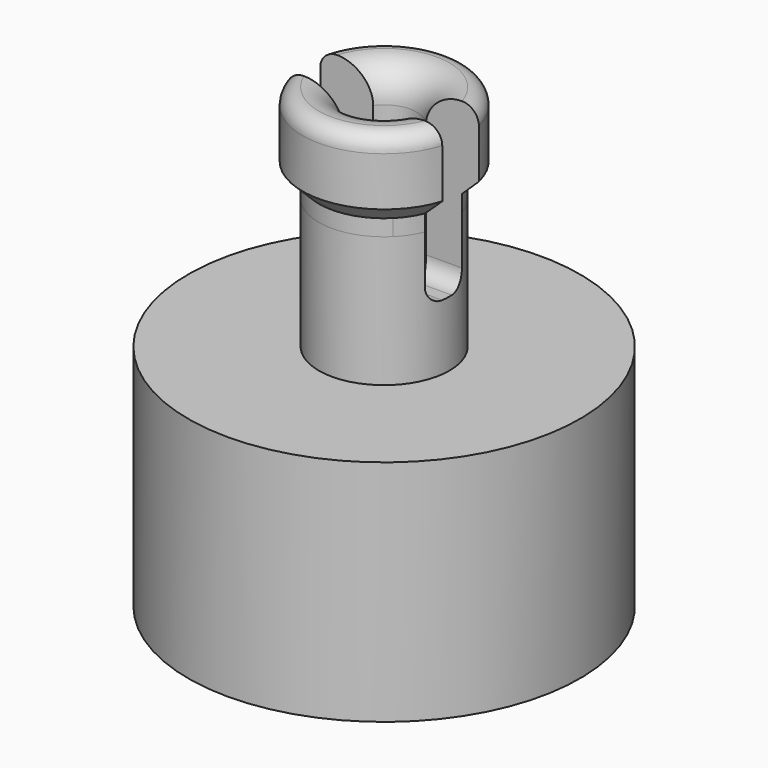
from build123d import *

# Parameters (mm, degrees)
F3_DEPTH     = 5
F4_T4_ANGLE  = 270.6670948428
F4_S5_R      = 2
F4_T6_DEPTH  = 5
F4_T10_ANGLE = 262.8807253971
F4_S11_R     = 2
F4_T12_DEPTH = 5
F5_SIZE      = 1
F6_R         = 1
F7_R         = 0.49999
F8_R         = 0.5
F9_W         = 20.6344220787
F9_H         = 19.8933202773
F9_R         = 5
F10_DEPTH    = 5
F11_R        = 2.8
F12_DEPTH    = 6.4


# Not quite as in the source:
# - a fillet or chamfer that OpenCascade refuses, or shapes differently, is made with other operations: its cross-section is extruded or revolved along the edge and cut away or added
# - a fillet or chamfer is up to 0.001 mm smaller than in the source, because OpenCascade refuses the exact size


with BuildPart() as f1:
    # F0 (on Right) → F1 (revolve)
    with BuildSketch(Plane.YZ):
        Polygon((-6, 0), (0, 0), (0, 12), (-1, 12), (-1, 16), (-1, 19), (-2, 19), (-2.5, 19), (-2.5, 16), (-2, 16), (-2, 12), (-6, 12), align=None)
    revolve(axis=Axis((0, 0, 6), (0, 0, -1)))

    # F2 (on face) → F3 (cut)
    with BuildSketch(Plane.XY.offset(19)):
        with BuildLine():
            Line((-0.8067003414, 0.5909607086), (-2.4291491187, 0.5909607086))
            ThreePointArc((-2.4291491187, 0.5909607086), (-2.4985623215, -0.0847721969), (-2.3835084063, -0.75424643))
            Line((-2.3835084063, -0.75424643), (-0.6565914428, -0.75424643))
            ThreePointArc((-0.6565914428, -0.75424643), (-0.993831612, -0.1108996261), (-0.8067003414, 0.5909607086))
        make_face()
        with BuildLine():
            ThreePointArc((1, 0), (0.9504473529, 0.3108855566), (0.8067003414, 0.5909607086))
            Line((0.8067003414, 0.5909607086), (-0.8067003414, 0.5909607086))
            ThreePointArc((-0.8067003414, 0.5909607086), (-0.993831612, -0.1108996261), (-0.6565914428, -0.75424643))
            Line((-0.6565914428, -0.75424643), (0.6565914428, -0.75424643))
            ThreePointArc((0.6565914428, -0.75424643), (0.9101075329, -0.4143721499), (1, 0))
        make_face()
        with BuildLine():
            ThreePointArc((2.5, 0), (2.482224083, 0.2975963737), (2.4291491187, 0.5909607086))
            Line((2.4291491187, 0.5909607086), (0.8067003414, 0.5909607086))
            ThreePointArc((0.8067003414, 0.5909607086), (0.9504473529, 0.3108855566), (1, 0))
            ThreePointArc((1, 0), (0.9101075329, -0.4143721499), (0.6565914428, -0.75424643))
            Line((0.6565914428, -0.75424643), (2.3835084063, -0.75424643))
            ThreePointArc((2.3835084063, -0.75424643), (2.4707054676, -0.38159467), (2.5, 0))
        make_face()
    extrude(amount=-F3_DEPTH, mode=Mode.SUBTRACT)

    # F4: chamfer of 1 on 2 edges, made by hand


with BuildPart() as f4_tool2:
    # F4_s3 → F4_t4 (revolve)
    with BuildSketch(Plane(origin=(0, 0, 0), x_dir=(0, 0, 1), z_dir=(0.7112111987, -0.7029784, 0))):
        Polygon((17, 2.5), (16, 1.5), (16, 2.5), align=None)
    revolve(axis=Axis((0, 0, 16), (0, 0, -1)), revolution_arc=F4_T4_ANGLE)

    # F4_s5 → F4_t6 (cut, symmetric)
    with BuildSketch(Plane.XY.offset(16.5)):
        Circle(F4_S5_R)
    extrude(amount=F4_T6_DEPTH, both=True, mode=Mode.SUBTRACT)


with BuildPart() as f1_1:
    add(f1.part)

    # F4_t1: cut F4_tool2
    add(f4_tool2.part, mode=Mode.SUBTRACT)


with BuildPart() as f4_tool8:
    # F4_s9 → F4_t10 (revolve)
    with BuildSketch(Plane(origin=(0, 0, 0), x_dir=(0, 0, 1), z_dir=(-0.6618401259, 0.7496450145, 0))):
        Polygon((17, 2.5), (16, 1.5), (16, 2.5), align=None)
    revolve(axis=Axis((0, 0, 16), (0, 0, -1)), revolution_arc=F4_T10_ANGLE)

    # F4_s11 → F4_t12 (cut, symmetric)
    with BuildSketch(Plane.XY.offset(16.5)):
        Circle(F4_S11_R)
    extrude(amount=F4_T12_DEPTH, both=True, mode=Mode.SUBTRACT)


with BuildPart() as f1_2:
    add(f1_1.part)

    # F4_t7: cut F4_tool8
    add(f4_tool8.part, mode=Mode.SUBTRACT)

    # F5
    f5_edges = [f1_2.edges().sort_by_distance(p)[0] for p in [
        (0, 6, 0),
    ]]
    chamfer(f5_edges, length=F5_SIZE)

    # F6
    f6_edges = [f1_2.edges().sort_by_distance(p)[0] for p in [
        (0, 1, 19),
        (-0.350538, -0.936549, 19),
        (0.350538, -0.936549, 19),
    ]]
    fillet(f6_edges, radius=F6_R)

    # F7 (radius 0.5 in the source; OpenCascade refuses exactly that, so slightly less here)
    f7_edges = [f1_2.edges().sort_by_distance(p)[0] for p in [
        (0, -2.5, 19),
        (0, 2.5, 19),
    ]]
    fillet(f7_edges, radius=F7_R)

    # F8
    f8_edges = [f1_2.edges().sort_by_distance(p)[0] for p in [
        (-1.254459, -0.754246, 14),
        (1.254459, -0.754246, 14),
        (-1.358699, 0.590961, 14),
        (1.358699, 0.590961, 14),
    ]]
    fillet(f8_edges, radius=F8_R)

    # F9 (on face) → F10 (cut)
    with BuildSketch(Plane(origin=(0, 0, 0), x_dir=(1, 0, 0), z_dir=(0, 0, -1))):
        with Locations((1.0028546676, -0.4471866414)):
            Rectangle(F9_W, F9_H)
        Circle(F9_R, mode=Mode.SUBTRACT)
        Circle(F9_R)
    extrude(amount=-F10_DEPTH, mode=Mode.SUBTRACT)

    # F11 (on face) → F12 (cut)
    with BuildSketch(Plane(origin=(0, 0, 5), x_dir=(1, 0, 0), z_dir=(0, 0, -1))):
        Circle(F11_R)
    extrude(amount=-F12_DEPTH, mode=Mode.SUBTRACT)


solid = f1_2.part
